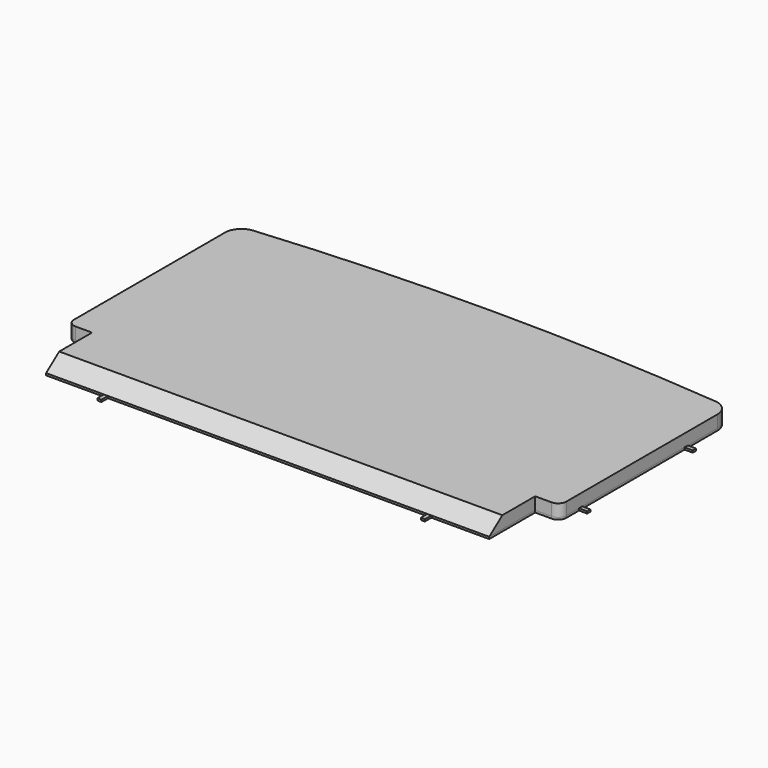
from build123d import *

# Parameters (mm, degrees)
F1_DEPTH = 19.05
F3_DEPTH = 723.901
F4_DEPTH = 3.175
F5_W     = 140.2353729725
F5_H     = 6.35
F5_W_2   = 6.35
F5_H_2   = 138.7533183813
F5_W_3   = 494.229254055
F5_H_3   = 197.8035473735
F6_DEPTH = 3.175


# Not quite as in the source:
# - a length typed as a fraction of an inch, garbled in the dataset ("3 / 203.2 mm" for 3/8 in), is restored


with BuildPart() as f1:
    # F0 (on Top) → F1 (new body)
    with BuildSketch(Plane.XY):
        with BuildLine():
            Line((38.1, 88.9), (38.1, 0))
            Line((38.1, 0), (723.9, 0))
            Line((723.9, 0), (723.9, 88.9))
            Line((723.9, 88.9), (749.3, 88.9))
            ThreePointArc((749.3, 88.9), (758.2802561211, 92.6197438789), (762, 101.6))
            Line((762, 101.6), (762, 393.7))
            ThreePointArc((762, 393.7), (755.3436522153, 410.8416306585), (738.8633463283, 418.9989577532))
            ThreePointArc((738.8633463283, 418.9989577532), (381, 434.975), (23.1366536717, 418.9989577532))
            ThreePointArc((23.1366536717, 418.9989577532), (6.6563477847, 410.8416306585), (0, 393.7))
            Line((0, 393.7), (0, 101.6))
            ThreePointArc((0, 101.6), (3.7197438789, 92.6197438789), (12.7, 88.9))
            Line((12.7, 88.9), (38.1, 88.9))
        make_face()
    extrude(amount=-F1_DEPTH)

    # F2 (on face) → F3 (cut, through all)
    with BuildSketch(Plane(origin=(38.1, 0, 0), x_dir=(0, -1, 0), z_dir=(-1, 0, 0))):
        Polygon((0, 0), (-25.4, 0), (0, -19.05), align=None)
    extrude(amount=-F3_DEPTH, mode=Mode.SUBTRACT)


with BuildPart() as f4:
    # F4 (new): a face of the model
    f4_faces = [f1.part.faces().sort_by_distance(p)[0] for p in [
        (381, 217.9962407233, -19.05),
    ]]
    extrude(f4_faces, amount=F4_DEPTH)

    # F5 (on face) → F6 (join)
    with BuildSketch(Plane(origin=(0, 0, -19.05), x_dir=(1, 0, 0), z_dir=(0, 0, -1))):
        with Locations((57.4176864862, -129.2283183813)):
            Rectangle(F5_W, F5_H)
        with Locations((130.7103729725, -56.6766591907)):
            Rectangle(F5_W_2, F5_H_2)
        with Locations((130.7103729725, -129.2283183813)):
            Rectangle(F5_W_2, F5_H)
        with Locations((381, -129.2283183813)):
            Rectangle(F5_W_3, F5_H)
        with Locations((130.7103729725, -231.3050920681)):
            Rectangle(F5_W_2, F5_H_3)
        with Locations((631.2896270275, -56.6766591907)):
            Rectangle(F5_W_2, F5_H_2)
        with Locations((631.2896270275, -129.2283183813)):
            Rectangle(F5_W_2, F5_H)
        Polygon((133.8853729725, -330.2068657549), (127.5353729725, -330.2068657549), (-12.7, -330.2068657549), (-12.7, -336.5568657549), (774.7, -336.5568657549), (774.7, -330.2068657549), (634.4646270275, -330.2068657549), (628.1146270275, -330.2068657549), align=None)
        with Locations((704.5823135138, -129.2283183813)):
            Rectangle(F5_W, F5_H)
        with Locations((631.2896270275, -231.3050920681)):
            Rectangle(F5_W_2, F5_H_3)
    extrude(amount=F6_DEPTH)


solid = Compound([f1.part, f4.part])
